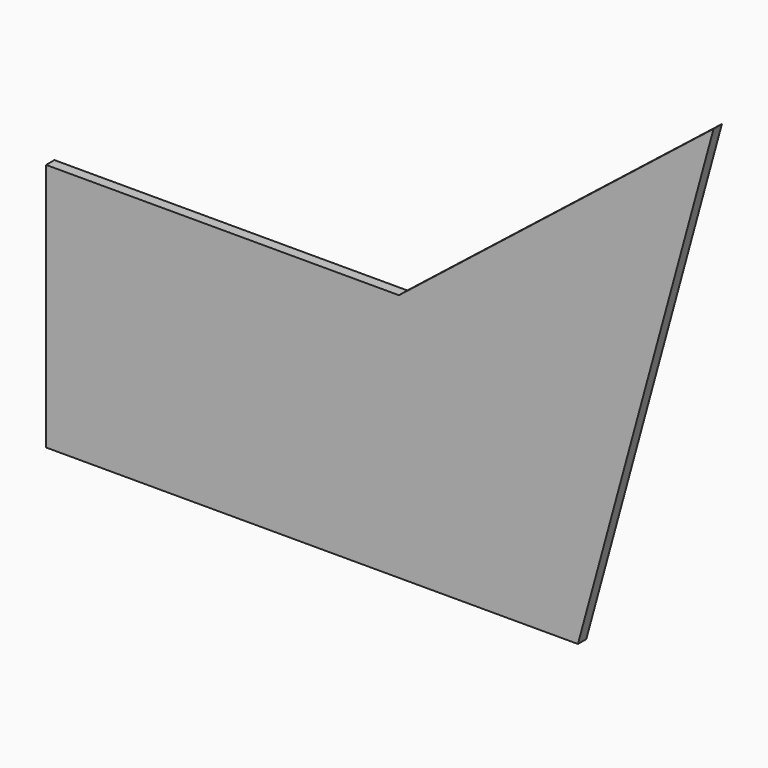
from build123d import *

# Parameters (mm, degrees)
F1_DEPTH = 2.38125


# Not quite as in the source:
# - a feature names something its author has since deleted; it is built from what else it names


with BuildPart() as f1:
    # F0 (on Front) → F1 (new body, symmetric)
    with BuildSketch(Plane.XZ):
        Polygon((-61.9342923164, 0), (0, 227.2394244377), (-143.6603479939, 113.6213351093), (-304.8, 113.6213351093), (-304.8, 0), align=None)
    extrude(amount=F1_DEPTH, both=True)


solid = f1.part
